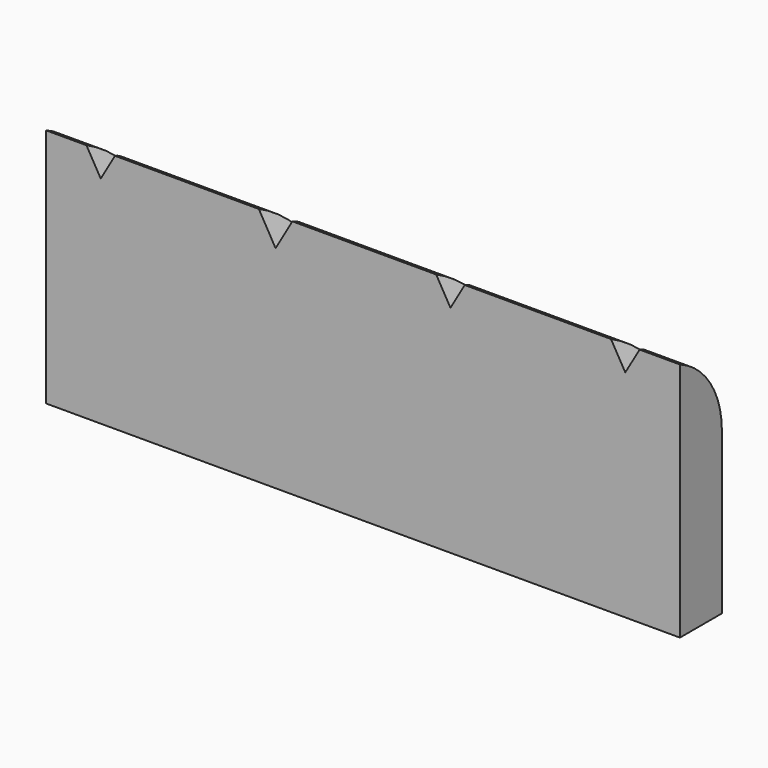
from build123d import *

# Parameters (mm, degrees)
F0_W        = 36.83
F0_H        = 3.048
F1_DEPTH    = 13.97
F3_T1_DEPTH = 60.1094845304
F4_DEPTH    = 25.4


# Not quite as in the source:
# - a fillet or chamfer that OpenCascade refuses, or shapes differently, is made with other operations: its cross-section is extruded or revolved along the edge and cut away or added


with BuildPart() as f1:
    # F0 (on Top) → F1 (new body)
    with BuildSketch(Plane.XY):
        with Locations((-0.254, 1.524)):
            Rectangle(F0_W, F0_H)
    extrude(amount=F1_DEPTH)

    # F3: fillet of radius 5.08 on 1 edges, made by hand

    # F3_s2 → F3_t1 (cut)
    with BuildSketch(Plane.YZ.offset(-30.3087422652)):
        with BuildLine():
            ThreePointArc((3.048, 9.3141030939), (2.2182329348, 12.0965336861), (0, 13.97))
            Line((0, 13.97), (3.048, 13.97))
            Line((3.048, 13.97), (3.048, 9.3141030939))
        make_face()
    extrude(amount=F3_T1_DEPTH, mode=Mode.SUBTRACT)

    # F2 (on face) → F4 (cut)
    with BuildSketch(Plane.XZ):
        Polygon((-15.494, 12.5322954744), (-14.6639409051, 13.97), (-16.3240590949, 13.97), align=None)
        Polygon((-4.3572939367, 13.97), (-6.3107060633, 13.97), (-5.334, 12.2782954744), align=None)
        Polygon((5.6560590949, 13.97), (3.9959409051, 13.97), (4.826, 12.5322954744), align=None)
        Polygon((15.8160590949, 13.97), (14.1559409051, 13.97), (14.986, 12.5322954744), align=None)
    extrude(amount=-F4_DEPTH, mode=Mode.SUBTRACT)


solid = f1.part
